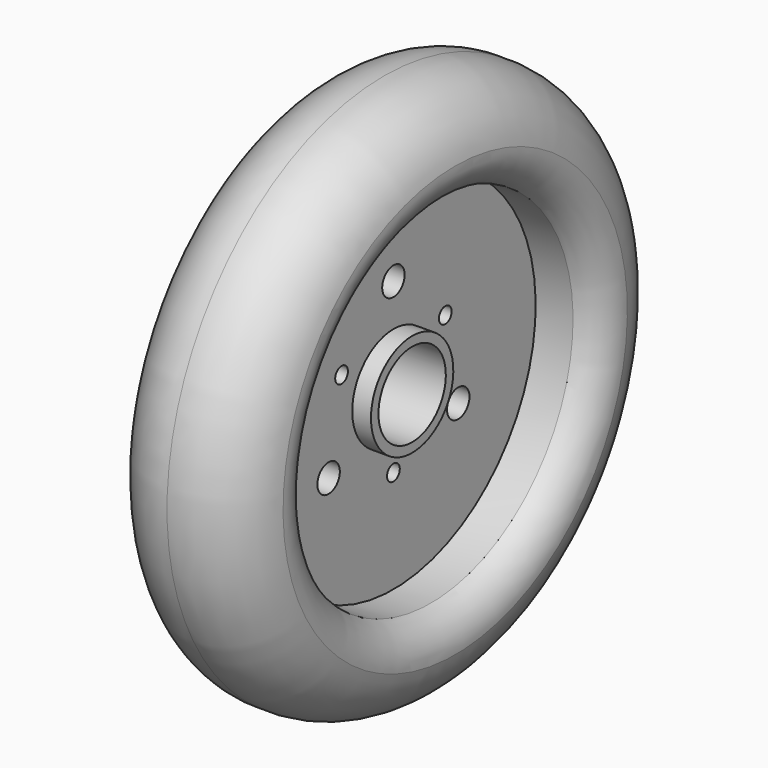
from build123d import *

# Parameters (mm, degrees)
F0_W           = 1
F0_H           = 1
F0_W_2         = 2
F0_H_2         = 13.5
F3_R           = 1.5
F3_R_2         = 0.85
F4_DEPTH       = 8.6165481942
F6_DEPTH       = 1.4
F7_R           = 3
F8_DEPTH       = 8
F9_R           = 4.2
F10_DEPTH      = 10.5
F11_R          = 7.4
F12_DEPTH      = 3.5
F13_R          = 5.6
F14_DEPTH      = 2
F15_R          = 1.5
F16_DEPTH      = 19.1165481942
F17_R          = 2
F18_DEPTH      = 7
F19_R          = 1.3
F20_DEPTH      = 6.5
F22_DEPTH      = 25
F22_DEPTH_BACK = 25


with BuildPart() as f2:
    # F0 (on Front) → F2 (revolve)
    with BuildSketch(Plane.XZ):
        with Locations((0.5, 5)):
            Rectangle(F0_W, F0_H)
        with Locations((-0.5, 5)):
            Rectangle(F0_W, F0_H)
        with Locations((2, 5)):
            Rectangle(F0_W_2, F0_H)
        with Locations((-0.5, 12.25)):
            Rectangle(F0_W, F0_H_2)
        with Locations((0.5, 12.25)):
            Rectangle(F0_W, F0_H_2)
        with Locations((-2, 5)):
            Rectangle(F0_W_2, F0_H)
        Polygon((0, 23), (0, 19), (1, 19), (5, 19), (5, 23), align=None)
        Polygon((-1, 19), (0, 19), (0, 23), (-5, 23), (-5, 19), align=None)
        with BuildLine():
            Line((-5, 23), (0, 23))
            Line((0, 23), (5, 23))
            Line((5, 23), (5, 19))
            ThreePointArc((5, 19), (6.9919404531, 20.5502387055), (7.6, 23))
            ThreePointArc((7.6, 23), (4.9375508317, 27.4408977202), (0, 29))
            ThreePointArc((0, 29), (-4.9375508317, 27.4408977202), (-7.6, 23))
            ThreePointArc((-7.6, 23), (-6.9919404531, 20.5502387055), (-5, 19))
            Line((-5, 19), (-5, 23))
        make_face()
    revolve(axis=Axis((4.0732044727, 0, 0), (1, 0, 0)))

    # F3 (on face) → F4 (cut, through all)
    with BuildSketch(Plane(origin=(-1, 0, 0), x_dir=(0, -1, 0), z_dir=(-1, 0, 0))):
        with Locations((0, 10)):
            Circle(F3_R)
        with Locations((-8.6602540378, -5)):
            Circle(F3_R)
        with Locations((8.6602540378, -5)):
            Circle(F3_R)
        with Locations((0, -8)):
            Circle(F3_R_2)
        with Locations((6.9282032303, 4)):
            Circle(F3_R_2)
        with Locations((-6.9282032303, 4)):
            Circle(F3_R_2)
    extrude(amount=-F4_DEPTH, mode=Mode.SUBTRACT)


with BuildPart() as f6:
    # F5 (on face) → F6 (new body)
    with BuildSketch(Plane(origin=(-1, 0, 0), x_dir=(0, -1, 0), z_dir=(-1, 0, 0))):
        with BuildLine():
            ThreePointArc((-4.3301270189, 12.5), (-1.2940952255, 5.1703708686), (5, 10))
            ThreePointArc((5, 10), (4.8296291314, 11.2940952255), (4.3301270189, 12.5))
            ThreePointArc((4.3301270189, 12.5), (0, 15), (-4.3301270189, 12.5))
        make_face()
        with BuildLine():
            ThreePointArc((4.3301270189, 12.5), (4.8296291314, 11.2940952255), (5, 10))
            ThreePointArc((5, 10), (-1.2940952255, 5.1703708686), (-4.3301270189, 12.5))
            Line((-4.3301270189, 12.5), (-12.9903810568, -2.5))
            ThreePointArc((-12.9903810568, -2.5), (-7.3661588123, -0.1703708686), (-3.6602540378, -5))
            ThreePointArc((-3.6602540378, -5), (-5.1247201319, -8.5355339059), (-8.6602540378, -10))
            Line((-8.6602540378, -10), (8.6602540378, -10))
            ThreePointArc((8.6602540378, -10), (4.3301270189, -2.5), (12.9903810568, -2.5))
            Line((12.9903810568, -2.5), (4.3301270189, 12.5))
        make_face()
        with BuildLine():
            ThreePointArc((13.6602540378, -5), (13.4898831693, -3.7059047745), (12.9903810568, -2.5))
            ThreePointArc((12.9903810568, -2.5), (4.3301270189, -2.5), (8.6602540378, -10))
            ThreePointArc((8.6602540378, -10), (12.1957879438, -8.5355339059), (13.6602540378, -5))
        make_face()
        with BuildLine():
            ThreePointArc((-3.6602540378, -5), (-7.3661588123, -0.1703708686), (-12.9903810568, -2.5))
            ThreePointArc((-12.9903810568, -2.5), (-12.9903810568, -7.5), (-8.6602540378, -10))
            ThreePointArc((-8.6602540378, -10), (-5.1247201319, -8.5355339059), (-3.6602540378, -5))
        make_face()
    extrude(amount=F6_DEPTH)

    # F7 (on face) → F8 (join)
    with BuildSketch(Plane.YZ.offset(-1)):
        with Locations((0, 10)):
            Circle(F7_R)
        with Locations((-8.6602540378, -5)):
            Circle(F7_R)
        with Locations((8.6602540378, -5)):
            Circle(F7_R)
    extrude(amount=-F8_DEPTH)

    # F9 (on face) → F10 (join)
    with BuildSketch(Plane.YZ.offset(-1)):
        Circle(F9_R)
    extrude(amount=-F10_DEPTH)

    # F11 (on face) → F12 (join)
    with BuildSketch(Plane.YZ.offset(-1)):
        Circle(F11_R)
    extrude(amount=-F12_DEPTH)

    # F13 (on face) → F14 (cut)
    with BuildSketch(Plane.YZ.offset(-1)):
        Circle(F13_R)
    extrude(amount=-F14_DEPTH, mode=Mode.SUBTRACT)

    # F15 (on face) → F16 (cut, through all)
    with BuildSketch(Plane(origin=(-11.5, 0, 0), x_dir=(0, -1, 0), z_dir=(-1, 0, 0))):
        Circle(F15_R)
    extrude(amount=-F16_DEPTH, mode=Mode.SUBTRACT)

    # F17 (on face) → F18 (cut)
    with BuildSketch(Plane(origin=(-11.5, 0, 0), x_dir=(0, -1, 0), z_dir=(-1, 0, 0))):
        Circle(F17_R)
    extrude(amount=-F18_DEPTH, mode=Mode.SUBTRACT)

    # F19 (on face) → F20 (cut)
    with BuildSketch(Plane.YZ.offset(-1)):
        with Locations((0, 10)):
            Circle(F19_R)
        with Locations((-8.6602540378, -5)):
            Circle(F19_R)
        with Locations((8.6602540378, -5)):
            Circle(F19_R)
    extrude(amount=-F20_DEPTH, mode=Mode.SUBTRACT)

    # F21 (on Front) → F22 (cut, two sides)
    with BuildSketch(Plane.XZ) as f22_sk:
        with BuildLine():
            Line((-11.5087675167, 1), (-11.5087675167, -1))
            Line((-11.5087675167, -1), (-9.5087675167, -1))
            ThreePointArc((-9.5087675167, -1), (-8.5087675167, 0), (-9.5087675167, 1))
            Line((-9.5087675167, 1), (-11.5087675167, 1))
        make_face()
    extrude(amount=-F22_DEPTH, mode=Mode.SUBTRACT)
    extrude(f22_sk.sketch, amount=F22_DEPTH_BACK, mode=Mode.SUBTRACT)


solid = Compound([f2.part, f6.part])
